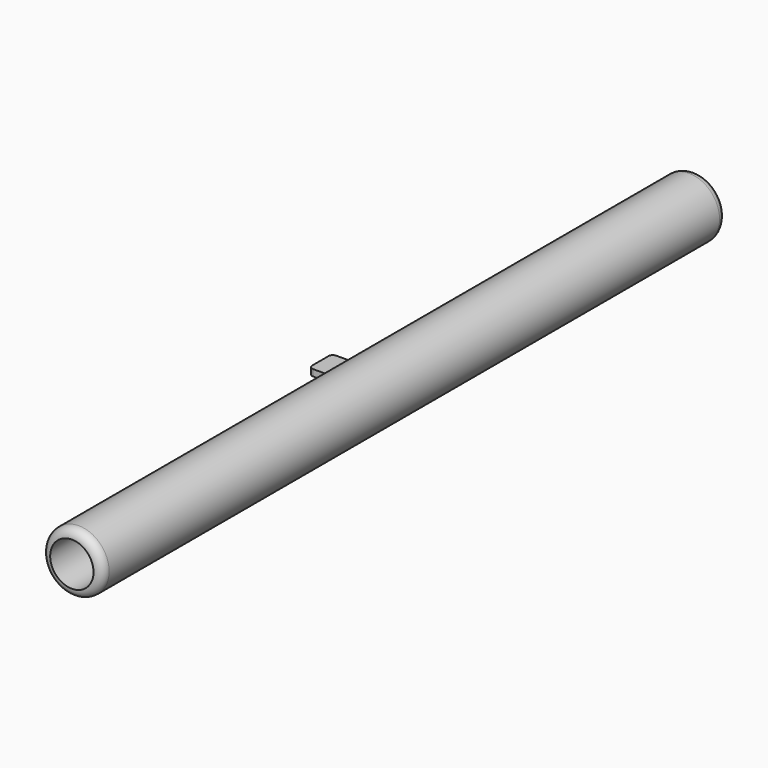
from build123d import *

# Parameters (mm, degrees)
F0_R     = 7
F0_R_2   = 5
F1_DEPTH = 90
F2_R     = 5
F3_DEPTH = 175
F4_R     = 1.99999
F6_DEPTH = 0.75
F7_R     = 1


# Not quite as in the source:
# - a fillet or chamfer is up to 0.001 mm smaller than in the source, because OpenCascade refuses the exact size


with BuildPart() as f1:
    # F0 (on Front) → F1 (new body, symmetric)
    with BuildSketch(Plane.XZ):
        Circle(F0_R)
        Circle(F0_R_2, mode=Mode.SUBTRACT)
        Circle(F0_R_2)
    extrude(amount=F1_DEPTH, both=True)

    # F2 (on face) → F3 (cut)
    with BuildSketch(Plane.XZ.offset(90)):
        Circle(F2_R)
    extrude(amount=-F3_DEPTH, mode=Mode.SUBTRACT)

    # F4 (radius 2 in the source; OpenCascade refuses exactly that, so slightly less here)
    f4_edges = [f1.edges().sort_by_distance(p)[0] for p in [
        (-7, 90, 0),
        (-7, -90, 0),
    ]]
    fillet(f4_edges, radius=F4_R)

    # F5 (on Top) → F6 (join, symmetric)
    with BuildSketch(Plane.XY):
        Polygon((-7, 0), (-7, 2.1346567392), (-13.7, 2.1346567392), (-13.7, -4.5653432608), (-7, -4.5653432608), align=None)
    extrude(amount=F6_DEPTH, both=True)

    # F7
    f7_edges = [f1.edges().sort_by_distance(p)[0] for p in [
        (-13.7, 2.134657, 0),
        (-13.7, -4.565343, 0),
    ]]
    fillet(f7_edges, radius=F7_R)


solid = f1.part
